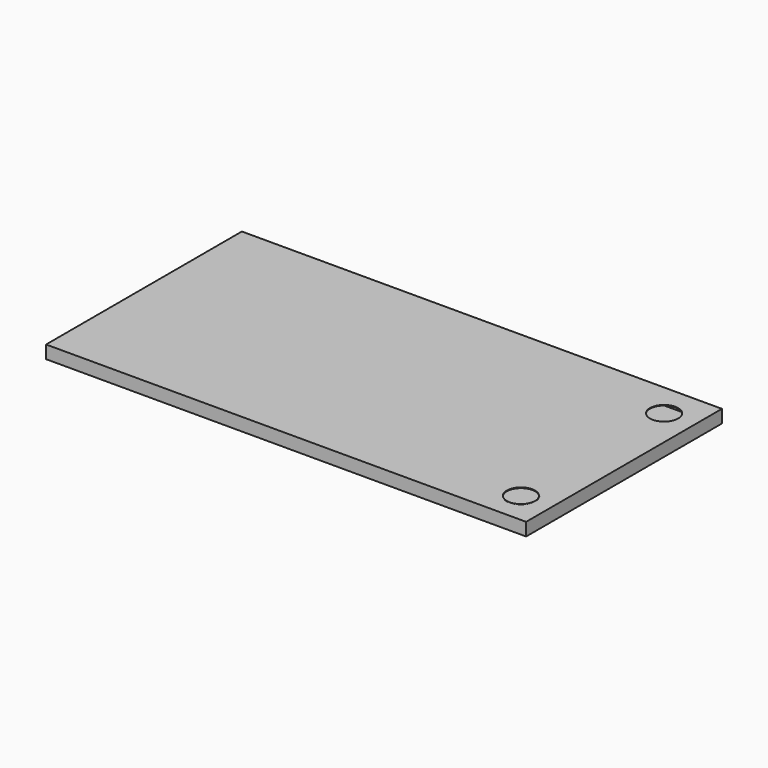
from build123d import *

# Parameters (mm, degrees)
F0_W     = 2040
F0_H     = 1040
F1_DEPTH = 50
F2_W     = 2040
F2_H     = 1040
F2_R     = 60
F3_DEPTH = 2.5
F4_W     = 2040
F4_H     = 1040
F5_DEPTH = 2.5
F6_R     = 61.25
F6_R_2   = 60
F7_DEPTH = 0.5


with BuildPart() as f1:
    # F0 (on Top) → F1 (new body)
    with BuildSketch(Plane.XY):
        Rectangle(F0_W, F0_H)
        Polygon((-1000, 250), (-1000, 500), (-750, 500), (1000, 500), (1000, 497.5), (1000, 250), (1000, -2.028e-07), (1000, -250), (1000, -497.5), (1000, -500), (-750, -500), (-1000, -500), (-1000, -250.0000003493), align=None, mode=Mode.SUBTRACT)
        with BuildLine():
            ThreePointArc((-750, -500), (-926.7766951731, -426.7766954201), (-1000, -250.0000003493))
            Line((-1000, -250.0000003493), (-1000, -500))
            Line((-1000, -500), (-750, -500))
        make_face()
        with BuildLine():
            ThreePointArc((-750, 0), (-926.7766952966, 73.2233047034), (-1000, 250))
            Line((-1000, 250), (-1000, -250.0000003493))
            ThreePointArc((-1000, -250.0000003493), (-926.7766954201, -73.2233048269), (-750, 0))
        make_face()
        with BuildLine():
            Line((-750, 500), (-1000, 500))
            Line((-1000, 500), (-1000, 250))
            ThreePointArc((-1000, 250), (-926.7766952966, 426.7766952966), (-750, 500))
        make_face()
        with BuildLine():
            Line((1000, -2.028e-07), (1000, 250))
            Line((1000, 250), (750, 250))
            ThreePointArc((750, 250), (926.7766953683, 176.7766952249), (1000, -2.028e-07))
        make_face()
        with BuildLine():
            Line((1000, -250), (1000, -2.028e-07))
            ThreePointArc((1000, -2.028e-07), (926.7766952249, -176.7766953683), (750, -250))
            Line((750, -250), (1000, -250))
        make_face()
        with BuildLine():
            ThreePointArc((750, -250), (926.7766952249, -176.7766953683), (1000, -2.028e-07))
            ThreePointArc((1000, -2.028e-07), (926.7766953683, 176.7766952249), (750, 250))
            Line((750, 250), (-750, 250))
            Line((-750, 250), (-750, 247.48))
            Line((-750, 247.48), (746.8536370203, 247.48))
            ThreePointArc((746.8536370203, 247.48), (997.4949999495, 1.5732132723), (750, -247.5))
            Line((750, -247.5), (-750, -247.5))
            Line((-750, -247.5), (-750, -250))
            Line((-750, -250), (750, -250))
        make_face()
        with BuildLine():
            Line((1000, 500), (-750, 500))
            ThreePointArc((-750, 500), (-926.7766952966, 426.7766952966), (-1000, 250))
            ThreePointArc((-1000, 250), (-926.7766952966, 73.2233047034), (-750, 0))
            ThreePointArc((-750, 0), (-926.7766954201, -73.2233048269), (-1000, -250.0000003493))
            ThreePointArc((-1000, -250.0000003493), (-926.7766951731, -426.7766954201), (-750, -500))
            Line((-750, -500), (1000, -500))
            Line((1000, -500), (1000, -497.5))
            Line((1000, -497.5), (-750, -497.5))
            ThreePointArc((-750, -497.5), (-997.5, -250), (-750, -2.5))
            Line((-750, -2.5), (750, -2.5))
            Line((750, -2.5), (750, 2.5))
            Line((750, 2.5), (-750, 2.5))
            ThreePointArc((-750, 2.5), (-997.5, 250), (-750, 497.5))
            Line((-750, 497.5), (1000, 497.5))
            Line((1000, 497.5), (1000, 500))
        make_face()
    extrude(amount=F1_DEPTH)

    # F2 (on face) → F3 (join)
    with BuildSketch(Plane.XY.offset(50)):
        Rectangle(F2_W, F2_H)
        with Locations((890, -385)):
            Circle(F2_R, mode=Mode.SUBTRACT)
        with Locations((890, 375)):
            Circle(F2_R, mode=Mode.SUBTRACT)
    extrude(amount=F3_DEPTH)

    # F4 (on face) → F5 (join)
    with BuildSketch(Plane(origin=(0, 0, 0), x_dir=(1, 0, 0), z_dir=(0, 0, -1))):
        Rectangle(F4_W, F4_H)
    extrude(amount=F5_DEPTH)

    # F6 (on face) → F7 (join)
    with BuildSketch(Plane.XY.offset(52.5)):
        with Locations((890, -385)):
            Circle(F6_R)
        with Locations((890, -385)):
            Circle(F6_R_2, mode=Mode.SUBTRACT)
    extrude(amount=F7_DEPTH)


solid = f1.part
